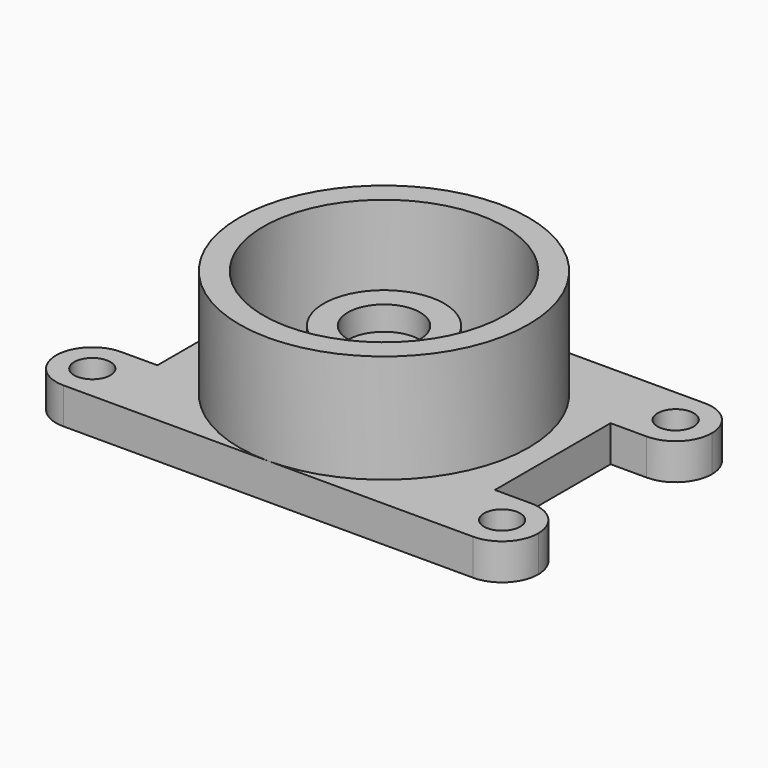
from build123d import *

# Parameters (mm, degrees)
F1_DEPTH  = 19.05
F0_R      = 63.5
F2_DEPTH  = 76.2
F0_R_2    = 31.75
F3_DEPTH  = 19.05
F0_R_3    = 19.05
F0_R_4    = 6.35
F4_DEPTH  = 50.8
F5_R      = 19.05
F6_DEPTH  = 12.7
F7_DEPTH  = 76.201
F8_DEPTH  = 19.05
F9_R      = 19.04999
F10_R     = 9.525
F11_DEPTH = 19.05


# Not quite as in the source:
# - a fillet or chamfer is up to 0.001 mm smaller than in the source, because OpenCascade refuses the exact size


with BuildPart() as f1:
    # F0 (on Top) → F1 (new body)
    with BuildSketch(Plane.XY):
        with BuildLine():
            ThreePointArc((0, 76.2), (53.8815367264, 53.8815367264), (76.2, 0))
            ThreePointArc((76.2, 0), (53.8815367264, -53.8815367264), (0, -76.2))
            Line((0, -76.2), (127, -76.2))
            Line((127, -76.2), (127, -38.1))
            Line((127, -38.1), (88.9, -38.1))
            Line((88.9, -38.1), (88.9, 38.1))
            Line((88.9, 38.1), (127, 38.1))
            Line((127, 38.1), (127, 76.2))
            Line((127, 76.2), (0, 76.2))
        make_face()
    extrude(amount=F1_DEPTH)

    # F0 (on Top) → F2 (join)
    with BuildSketch(Plane.XY):
        with BuildLine():
            ThreePointArc((0, -76.2), (53.8815367264, -53.8815367264), (76.2, 0))
            ThreePointArc((76.2, 0), (53.8815367264, 53.8815367264), (0, 76.2))
            ThreePointArc((0, 76.2), (-76.2, 0), (0, -76.2))
        make_face()
        Circle(F0_R, mode=Mode.SUBTRACT)
    extrude(amount=F2_DEPTH)

    # F0 (on Top) → F3 (join)
    with BuildSketch(Plane.XY):
        Circle(F0_R)
        Circle(F0_R_2, mode=Mode.SUBTRACT)
    extrude(amount=F3_DEPTH)

    # F0 (on Top) → F4 (join)
    with BuildSketch(Plane.XY):
        Circle(F0_R_2)
        Circle(F0_R_3, mode=Mode.SUBTRACT)
        Circle(F0_R_3)
        Circle(F0_R_4, mode=Mode.SUBTRACT)
        Circle(F0_R_4)
    extrude(amount=F4_DEPTH)

    # F5 (on face) → F6 (cut)
    with BuildSketch(Plane.XY.offset(50.8)):
        Circle(F5_R)
    extrude(amount=-F6_DEPTH, mode=Mode.SUBTRACT)

    # F0 (on Top) → F7 (cut, through all)
    with BuildSketch(Plane.XY):
        Circle(F0_R_4)
    extrude(amount=F7_DEPTH, mode=Mode.SUBTRACT)

    # F0 (on Top) → F8 (join)
    with BuildSketch(Plane.XY):
        with BuildLine():
            ThreePointArc((0, -76.2), (-76.2, 0), (0, 76.2))
            Line((0, 76.2), (-127, 76.2))
            Line((-127, 76.2), (-127, 38.1))
            Line((-127, 38.1), (-88.9, 38.1))
            Line((-88.9, 38.1), (-88.9, -38.1))
            Line((-88.9, -38.1), (-127, -38.1))
            Line((-127, -38.1), (-127, -76.2))
            Line((-127, -76.2), (0, -76.2))
        make_face()
    extrude(amount=F8_DEPTH)

    # F9 (radius 19.05 in the source; OpenCascade refuses exactly that, so slightly less here)
    f9_edges = [f1.edges().sort_by_distance(p)[0] for p in [
        (-127, -76.2, 9.525),
        (-127, -38.1, 9.525),
        (-127, 38.1, 9.525),
        (-127, 76.2, 9.525),
        (127, 38.1, 9.525),
        (127, 76.2, 9.525),
        (127, -76.2, 9.525),
        (127, -38.1, 9.525),
    ]]
    fillet(f9_edges, radius=F9_R)

    # F10 (on face) → F11 (cut, through all)
    with BuildSketch(Plane.XY.offset(19.05)):
        with Locations((-107.95, -57.15)):
            Circle(F10_R)
        with Locations((-107.95, 57.15)):
            Circle(F10_R)
        with Locations((107.95, 57.15)):
            Circle(F10_R)
        with Locations((107.95, -57.15)):
            Circle(F10_R)
    extrude(amount=-F11_DEPTH, mode=Mode.SUBTRACT)


solid = f1.part
